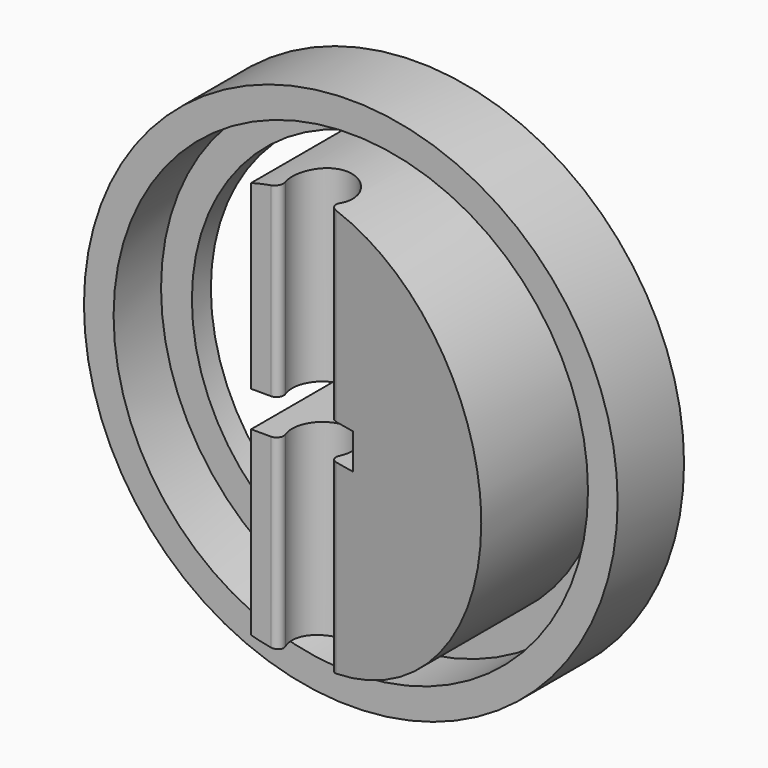
from build123d import *

# Parameters (mm, degrees)
F0_R           = 28.575
F1_DEPTH       = 8.89
F2_R           = 25.4
F3_DEPTH       = 6.35
F4_R           = 22.098
F5_DEPTH       = 10.16
F5_DEPTH_BACK  = 6.35
F7_DEPTH       = 84
F8_R           = 0.762
F10_DEPTH      = 14.9298409544
F11_W          = 11.43
F11_H          = 3.81
F12_DEPTH      = 6.35
F12_DEPTH_BACK = 10.1610001


# Not quite as in the source:
# - an extrude ends at something that could not be found from the text; its depth is read off the source's solid
# - a pattern or mirror of a feature is missing from the dataset's text; its kind, count and spacing are read off the source's solid


with BuildPart() as f1:
    # F0 (on Front) → F1 (new body)
    with BuildSketch(Plane.XZ):
        Circle(F0_R)
    extrude(amount=-F1_DEPTH)

    # F2 (on face) → F3 (cut)
    with BuildSketch(Plane.XZ):
        Circle(F2_R)
    extrude(amount=-F3_DEPTH, mode=Mode.SUBTRACT)

    # F4 (on face) → F5 (join, two sides)
    with BuildSketch(Plane.XZ) as f5_sk:
        Circle(F4_R)
    extrude(amount=F5_DEPTH)
    extrude(f5_sk.sketch, amount=-F5_DEPTH_BACK)

    # F6 (on Top) → F7 (cut, through all)
    with BuildSketch(Plane.XY):
        with BuildLine():
            Line((-23.6465651542, -10.16), (22.098, -10.16))
            Line((22.098, -10.16), (2.3495, -6.0388409544))
            ThreePointArc((2.3495, -6.0388409544), (0, -0.5715), (-2.3495, -6.0388409544))
            Line((-2.3495, -6.0388409544), (-23.6465651542, -6.0388409544))
            Line((-23.6465651542, -6.0388409544), (-23.6465651542, -10.16))
        make_face()
    f7 = extrude(amount=-F7_DEPTH, mode=Mode.SUBTRACT)

    # F7_copies: F7 across plane
    add(f7.mirror(Plane.XY), mode=Mode.SUBTRACT)

    # F8
    f8_edges = [f1.edges().sort_by_distance(p)[0] for p in [
        (-2.3495, -6.038841, 0),
        (2.3495, -6.038841, 0),
    ]]
    fillet(f8_edges, radius=F8_R)

    # F9 (on face) → F10 (cut, through all)
    with BuildSketch(Plane.XZ.offset(6.0388409544)):
        with BuildLine():
            Line((-5.842, -21.3117957948), (-5.842, 21.3117957948))
            ThreePointArc((-5.842, 21.3117957948), (-22.098, 0), (-5.842, -21.3117957948))
        make_face()
    extrude(amount=-F10_DEPTH, mode=Mode.SUBTRACT)

    # F11 (on Front) → F12 (cut, two sides)
    with BuildSketch(Plane.XZ) as f12_sk:
        with Locations((-0.127, 0)):
            Rectangle(F11_W, F11_H)
    extrude(amount=-F12_DEPTH, mode=Mode.SUBTRACT)
    extrude(f12_sk.sketch, amount=F12_DEPTH_BACK, mode=Mode.SUBTRACT)


solid = f1.part
